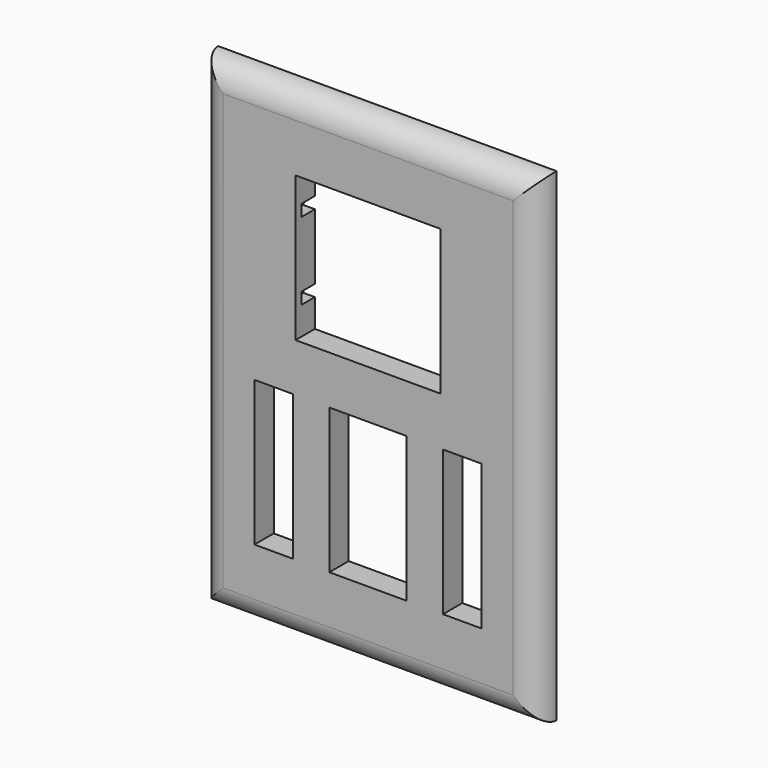
from build123d import *

# Parameters (mm, degrees)
F0_W      = 88.9
F0_H      = 127
F1_DEPTH  = 6.35
F2_R      = 6.34999
F3_W      = 38.1
F3_H      = 38.1
F4_DEPTH  = 6.351
F5_W      = 20.32
F5_H      = 38.1
F5_W_2    = 10.16
F6_DEPTH  = 6.351
F7_W      = 4.318
F7_H      = 3.048
F8_DEPTH  = 3.048
F9_W      = 4.318
F9_H      = 3.048
F10_DEPTH = 3.048


# Not quite as in the source:
# - a fillet or chamfer is up to 0.001 mm smaller than in the source, because OpenCascade refuses the exact size


with BuildPart() as f1:
    # F0 (on Front) → F1 (new body)
    with BuildSketch(Plane.XZ):
        Rectangle(F0_W, F0_H)
    extrude(amount=F1_DEPTH)

    # F2 (radius 6.35 in the source; OpenCascade refuses exactly that, so slightly less here)
    f2_edges = [f1.edges().sort_by_distance(p)[0] for p in [
        (-44.45, -6.35, 0),
        (0, -6.35, 63.5),
        (44.45, -6.35, 0),
        (0, -6.35, -63.5),
    ]]
    fillet(f2_edges, radius=F2_R)

    # F3 (on face) → F4 (cut, through all)
    with BuildSketch(Plane.XZ.offset(6.35)):
        with Locations((0, 25.4)):
            Rectangle(F3_W, F3_H)
    extrude(amount=-F4_DEPTH, mode=Mode.SUBTRACT)

    # F5 (on face) → F6 (cut, through all)
    with BuildSketch(Plane.XZ.offset(6.35)):
        with Locations((0, -25.4)):
            Rectangle(F5_W, F5_H)
        with Locations((-24.765, -25.4)):
            Rectangle(F5_W_2, F5_H)
        with Locations((24.765, -25.4)):
            Rectangle(F5_W_2, F5_H)
    extrude(amount=-F6_DEPTH, mode=Mode.SUBTRACT)

    # F7 (on face) → F8 (cut)
    with BuildSketch(Plane.YZ.offset(-19.05)):
        with Locations((-2.159, 35.56)):
            Rectangle(F7_W, F7_H)
        with Locations((-2.159, 15.24)):
            Rectangle(F7_W, F7_H)
    extrude(amount=-F8_DEPTH, mode=Mode.SUBTRACT)

    # F9 (on face) → F10 (cut)
    with BuildSketch(Plane(origin=(19.05, 0, 0), x_dir=(0, -1, 0), z_dir=(-1, 0, 0))):
        with Locations((2.159, 15.24)):
            Rectangle(F9_W, F9_H)
        with Locations((2.159, 35.56)):
            Rectangle(F9_W, F9_H)
    extrude(amount=-F10_DEPTH, mode=Mode.SUBTRACT)


solid = f1.part
